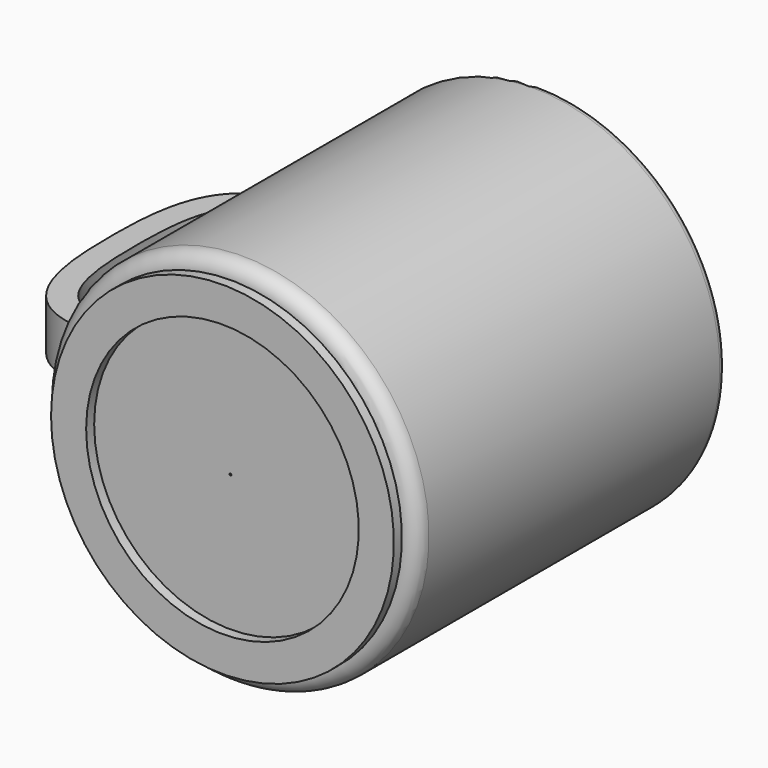
from build123d import *

# Parameters (mm, degrees)
F4_DEPTH = 10


# Not quite as in the source:
# - ends of sketch curves that miss each other by under 0.0002 mm in the source are joined
# - the dataset's text gives a spline's control points without its knots; the knots are read off the source's solid


with BuildPart() as f2:
    # F0 (on Top) → F2 (revolve)
    with BuildSketch(Plane.XY):
        with BuildLine():
            ThreePointArc((-30.7526913285, 40.8521510884), (-31.8133515003, 40.4128112602), (-32.2526913285, 39.3521510884))
            Line((-32.2526913285, 39.3521510884), (-32.2526913285, -33.1478489116))
            ThreePointArc((-32.2526913285, -33.1478489116), (-31.3740116721, -35.2691692551), (-29.2526913285, -36.1478489116))
            Line((-29.2526913285, -36.1478489116), (-29.2526913285, -38.1478489116))
            Line((-29.2526913285, -38.1478489116), (-22.2526913285, -38.1478489116))
            Line((-22.2526913285, -38.1478489116), (-22.2526913285, -36.1478489116))
            Line((-22.2526913285, -36.1478489116), (4.7473086715, -36.1478489116))
            Line((4.7473086715, -36.1478489116), (4.7473086715, -29.1478489116))
            Line((4.7473086715, -29.1478489116), (-22.2526913285, -29.1478489116))
            ThreePointArc((-22.2526913285, -29.1478489116), (-24.3740116721, -28.2691692551), (-25.2526913285, -26.1478489116))
            Line((-25.2526913285, -26.1478489116), (-25.2526913285, 40.8521510884))
            Line((-25.2526913285, 40.8521510884), (-30.7526913285, 40.8521510884))
        make_face()
    revolve(axis=Axis((4.9331779592, -31.1005194671, 0), (0, -1, 0)))

    # F3 (on Top) → F4 (join)
    with BuildSketch(Plane.XY):
        with BuildLine():
            Line((-32.3123847502, 22.2678844626), (-32.2659313679, 27.3156445473))
            add(Edge.make_bspline(
                [(-32.2659313679, 27.3156445473), (-46.6006913711, 25.6773854639), (-49.0956164188, 0.3705835796), (-46.6173155902, -26.2457033085), (-32.25120157, -27.0666256547)],
                knots=[0, 0, 0, 0, 0.5008322198, 1, 1, 1, 1], degree=3))
            Line((-32.25120157, -27.0666256547), (-32.3309251315, -22.0502301452))
            add(Edge.make_bspline(
                [(-32.3123847502, 22.2678844626), (-33.4716919712, 22.0974672329), (-35.0256169178, 21.6894005601), (-36.65466392, 20.9370544367), (-37.7430115827, 20.2279217443), (-38.6665983287, 19.4104966031), (-39.4758862474, 18.4569944727), (-40.1960390774, 17.3365367297), (-41.044620924, 15.5946549331), (-41.8842799371, 12.937926474), (-42.4088463082, 9.7295553854), (-42.6626364808, 6.9190082723), (-42.7815080406, 4.7102652819), (-42.8315091709, 2.8021541851), (-42.8493277453, 1.2455509128), (-42.8534876415, 0.0630161959), (-42.8505277309, -1.1231769809), (-42.8346125599, -2.6886700722), (-42.7872915368, -4.6168578294), (-42.6717858521, -6.8602755709), (-42.4220686001, -9.7269871551), (-41.9006891843, -13.0153991581), (-41.0593415398, -15.7357819013), (-40.2130595814, -17.4953559245), (-39.5015471065, -18.6072874524), (-38.713776754, -19.52877869), (-37.8283504544, -20.2943792449), (-36.791909777, -20.9386340193), (-35.5278061858, -21.4736451512), (-34.0510409441, -21.8555480747), (-32.8968655243, -22.0063328549), (-32.3309251315, -22.0502301452)],
                knots=[0.0091708789, 0.0091708789, 0.0091708789, 0.0091708789, 0.0625, 0.09375, 0.125, 0.15625, 0.1875, 0.21875, 0.25, 0.3125, 0.375, 0.40625, 0.4375, 0.46875, 0.484375, 0.5, 0.515625, 0.53125, 0.5625, 0.59375, 0.625, 0.6875, 0.75, 0.78125, 0.8125, 0.84375, 0.875, 0.90625, 0.9375, 0.96875, 0.9945451461, 0.9945451461, 0.9945451461, 0.9945451461], degree=3))
        make_face()
    extrude(amount=F4_DEPTH)


solid = f2.part
